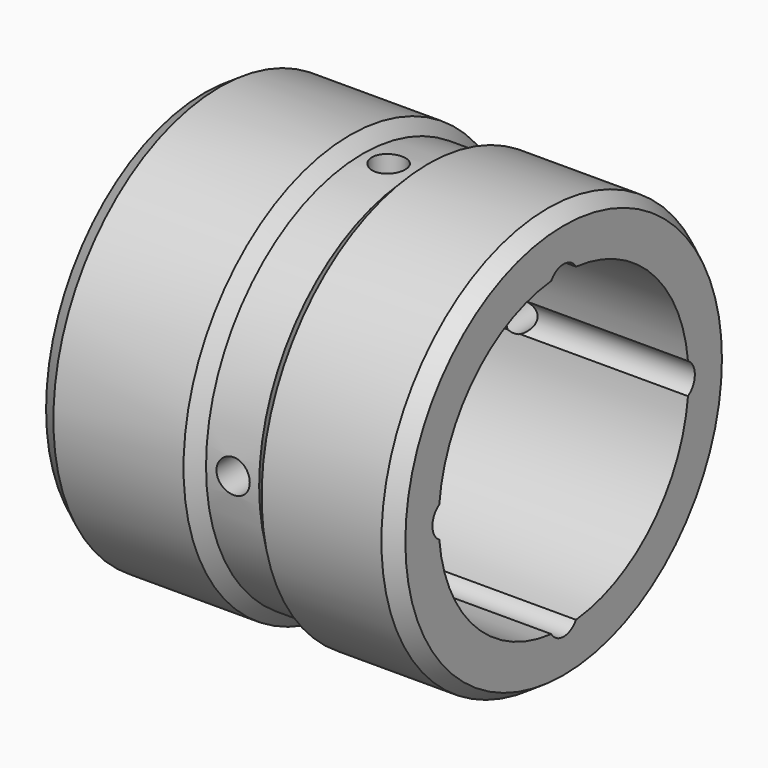
from build123d import *

# Parameters (mm, degrees)
F2_R          = 1.75
F3_DEPTH      = 34.501
F4_R          = 1.6
F5_DEPTH      = 20.001
F5_DEPTH_BACK = 20.001
F6_R          = 1.6
F7_DEPTH      = 20.001
F7_DEPTH_BACK = 20.001
F8_C1_SIZE2   = 1.5
F8_C1_SIZE    = 1
F8_C2_SIZE2   = 1.5
F8_C2_SIZE    = 1


# Not quite as in the source:
# - two fillets or chamfers of one size are made in one step


with BuildPart() as f1:
    # F0 (on Front) → F1 (revolve)
    with BuildSketch(Plane.XZ):
        Polygon((0, 20), (0, 15), (34.5, 15), (34.5, 20), (21.5, 20), (20.3, 18.8), (15.2, 18.8), (14, 20), align=None)
    revolve(axis=Axis((0.4285710554, 0, 0), (1, 0, 0)))

    # F2 (on Right) → F3 (cut, through all)
    with BuildSketch(Plane.YZ):
        with Locations((14, 0)):
            Circle(F2_R)
        with Locations((0, 14)):
            Circle(F2_R)
        with Locations((-14, 0)):
            Circle(F2_R)
        with Locations((0, -14)):
            Circle(F2_R)
    extrude(amount=F3_DEPTH, mode=Mode.SUBTRACT)

    # F4 (on Top) → F5 (cut, two sides)
    with BuildSketch(Plane.XY) as f5_sk:
        with Locations((17.7, 0)):
            Circle(F4_R)
    extrude(amount=-F5_DEPTH, mode=Mode.SUBTRACT)
    extrude(f5_sk.sketch, amount=F5_DEPTH_BACK, mode=Mode.SUBTRACT)

    # F6 (on Front) → F7 (cut, two sides)
    with BuildSketch(Plane.XZ) as f7_sk:
        with Locations((17.8, 0)):
            Circle(F6_R)
    extrude(amount=-F7_DEPTH, mode=Mode.SUBTRACT)
    extrude(f7_sk.sketch, amount=F7_DEPTH_BACK, mode=Mode.SUBTRACT)

    # F8: chamfer of 1.5 x 1 on 2 edges, made by hand

    # F8_c1
    f8_c1_edges = [f1.edges().sort_by_distance(p)[0] for p in [
        (0, 0, -20),
    ]]
    f8_c1_side = f1.faces().sort_by_distance((0, 0, -19.98))[0]
    chamfer(f8_c1_edges, length=F8_C1_SIZE, length2=F8_C1_SIZE2, reference=f8_c1_side)

    # F8_c2
    f8_c2_edges = [f1.edges().sort_by_distance(p)[0] for p in [
        (34.5, 0, -20),
    ]]
    f8_c2_side = f1.faces().sort_by_distance((34.5, 0, -19.98))[0]
    chamfer(f8_c2_edges, length=F8_C2_SIZE, length2=F8_C2_SIZE2, reference=f8_c2_side)


solid = f1.part
